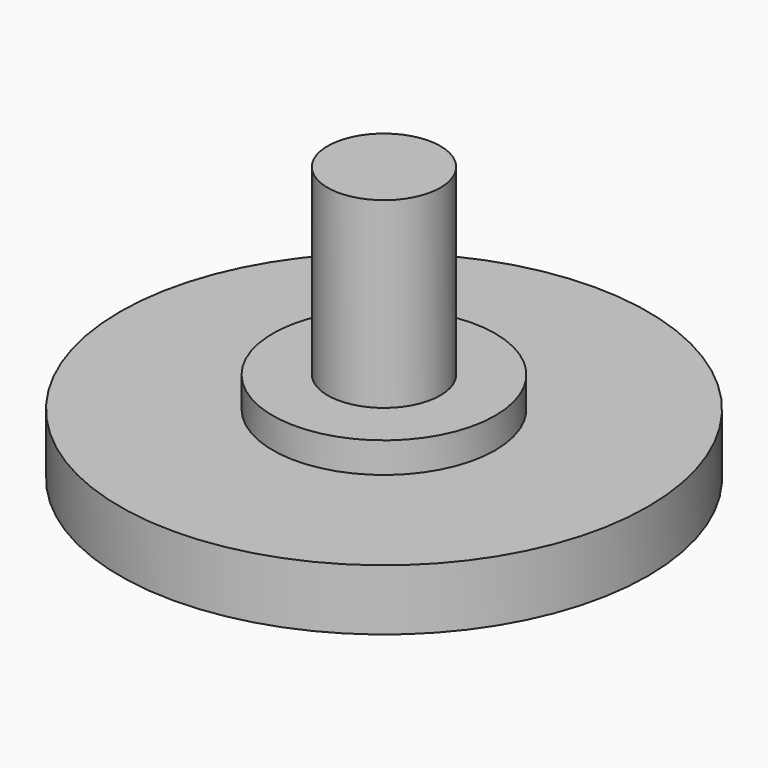
from build123d import *

# Parameters (mm, degrees)
F0_R     = 2.35
F1_DEPTH = 11.43
F0_R_2   = 4.636
F2_DEPTH = 3.81
F0_R_3   = 11
F3_DEPTH = 2.54
F5_DEPTH = 1.27
F6_R     = 1.26999


# Not quite as in the source:
# - a fillet or chamfer is up to 0.001 mm smaller than in the source, because OpenCascade refuses the exact size


with BuildPart() as f1:
    # F0 (on Top) → F1 (new body)
    with BuildSketch(Plane.XY):
        Circle(F0_R)
    extrude(amount=F1_DEPTH)

    # F0 (on Top) → F2 (join)
    with BuildSketch(Plane.XY):
        Circle(F0_R_2)
        Circle(F0_R, mode=Mode.SUBTRACT)
    extrude(amount=F2_DEPTH)

    # F0 (on Top) → F3 (join)
    with BuildSketch(Plane.XY):
        Circle(F0_R_3)
        Circle(F0_R_2, mode=Mode.SUBTRACT)
    extrude(amount=F3_DEPTH)

    # F4 (on face) → F5 (join)
    with BuildSketch(Plane.XY):
        with BuildLine():
            Line((-5.0818, -4.396), (-5.0818, -7.19))
            Line((-5.0818, -7.19), (5.0782, -7.19))
            Line((5.0782, -7.19), (5.0782, -4.396))
            Line((5.0782, -4.396), (2.0302, -4.396))
            ThreePointArc((2.0302, -4.396), (1.611480541, 0.7864996759), (-2.0338, 4.494))
            ThreePointArc((-2.0338, 4.494), (-0.603014409, 0.049), (-2.0338, -4.396))
            Line((-2.0338, -4.396), (-5.0818, -4.396))
        make_face()
    extrude(amount=-F5_DEPTH)

    # F6 (radius 1.27 in the source; OpenCascade refuses exactly that, so slightly less here)
    f6_edges = [f1.edges().sort_by_distance(p)[0] for p in [
        (5.0782, -5.793, -1.27),
        (-5.0818, -5.793, -1.27),
        (-0.0018, -7.19, -1.27),
        (-3.5578, -4.396, -1.27),
        (3.5542, -4.396, -1.27),
        (1.611481, 0.7865, -1.27),
        (-0.603014, 0.049, -1.27),
    ]]
    fillet(f6_edges, radius=F6_R)


solid = f1.part
